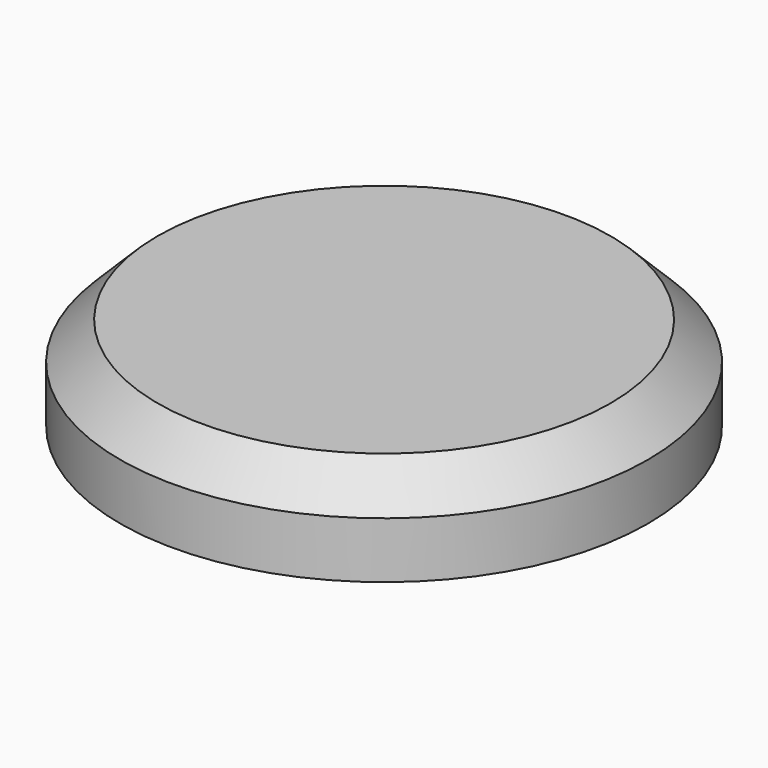
from build123d import *

# Parameters (mm, degrees)
F0_R     = 35.7733555676
F1_DEPTH = 12.7
F2_SIZE  = 5.08


# Not quite as in the source:
# - the program builds the solid bodies; features that only make, move or delete a surface that nothing else refers to are left out


with BuildPart() as f1:
    # F0 (on Top) → F1 (new body)
    with BuildSketch(Plane.XY):
        Circle(F0_R)
    extrude(amount=F1_DEPTH)

    # F2
    f2_edges = [f1.edges().sort_by_distance(p)[0] for p in [
        (-35.773356, 0, 12.7),
    ]]
    chamfer(f2_edges, length=F2_SIZE)


solid = f1.part
